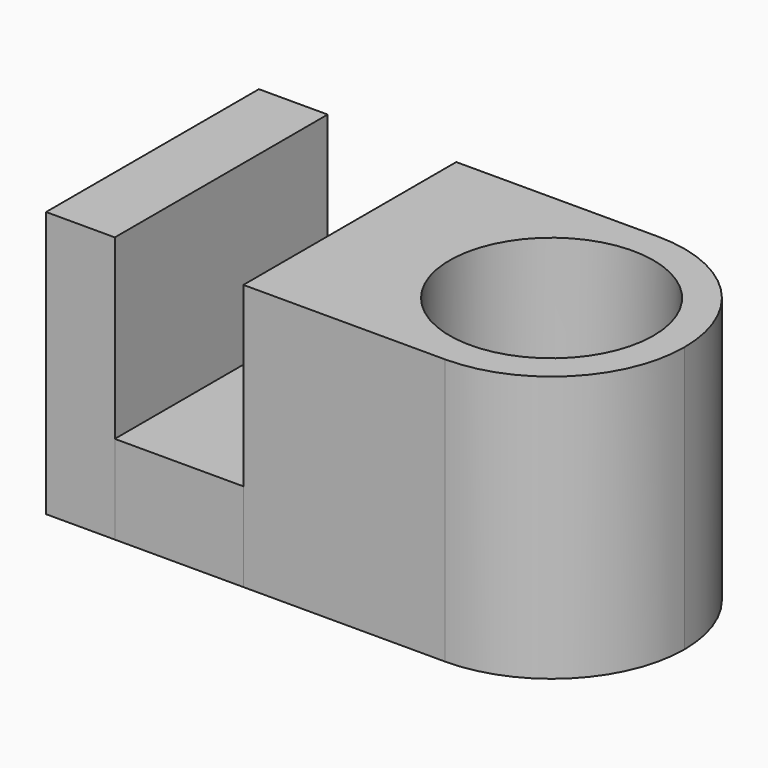
from build123d import *

# Parameters (mm, degrees)
F0_W     = 30
F0_H     = 30
F0_R     = 11.5
F1_DEPTH = 30
F0_W_2   = 7.75
F2_DEPTH = 30
F0_W_3   = 14.5
F3_DEPTH = 10
F4_R     = 14.99999


# Not quite as in the source:
# - a fillet or chamfer is up to 0.001 mm smaller than in the source, because OpenCascade refuses the exact size


with BuildPart() as f1:
    # F0 (on Top) → F1 (new body)
    with BuildSketch(Plane.XY):
        with Locations((15, 0)):
            Rectangle(F0_W, F0_H)
        with Locations((15, 0)):
            Circle(F0_R, mode=Mode.SUBTRACT)
    extrude(amount=F1_DEPTH)

    # F0 (on Top) → F2, piece 2 (join)
    with BuildSketch(Plane.XY):
        with Locations((-3.875, 0)):
            Rectangle(F0_W_2, F0_H)
    extrude(amount=F2_DEPTH)

    # F4 (radius 15 in the source; OpenCascade refuses exactly that, so slightly less here)
    f4_edges = [f1.edges().sort_by_distance(p)[0] for p in [
        (30, -15, 15),
        (30, 15, 15),
    ]]
    fillet(f4_edges, radius=F4_R)


with BuildPart() as f2:
    # F0 (on Top) → F2 (new body)
    with BuildSketch(Plane.XY):
        with Locations((-26.125, 0)):
            Rectangle(F0_W_2, F0_H)
    extrude(amount=F2_DEPTH)


with BuildPart() as f3:
    # F0 (on Top) → F3 (new body)
    with BuildSketch(Plane.XY):
        with Locations((-15, 0)):
            Rectangle(F0_W_3, F0_H)
    extrude(amount=F3_DEPTH)


solid = Compound([f1.part, f2.part, f3.part])
